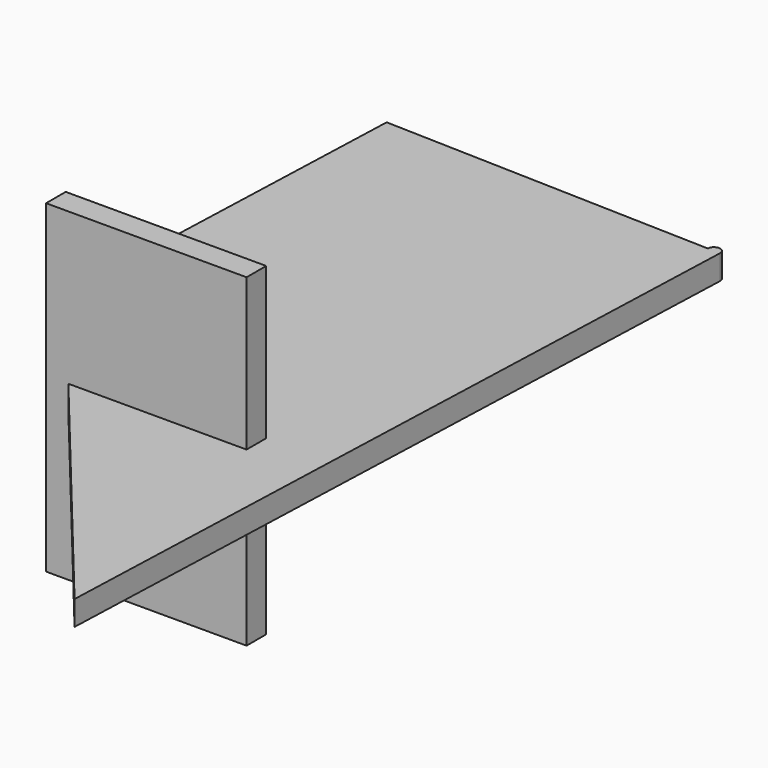
from build123d import *

# Parameters (mm, degrees)
F2_DEPTH = 25
F3_W     = 204.2875885963
F3_H     = 330.4814696312
F4_DEPTH = 25


with BuildPart() as f2:
    # F1 (on Top) → F2 (new body)
    with BuildSketch(Plane.XY):
        with BuildLine():
            Line((168.3422140292, 474.8379558081), (181.0361660289, 474.454610266))
            ThreePointArc((181.0361660289, 474.454610266), (174.8820955467, 481.0340797179), (168.3422140292, 474.8379558081))
        make_face()
        with BuildLine():
            Line((166.6445245232, 81.42426457), (181.0361660289, 474.454610266))
            Line((181.0361660289, 474.454610266), (168.3422140292, 474.8379558081))
            Line((168.3422140292, 474.8379558081), (-166.9943213011, 484.9648072356))
            Line((-166.9943213011, 484.9648072356), (-178.021518384, 183.8161801091))
            add(Edge.make_bspline(
                [(-178.021518384, 183.8161801091), (-126.121723234, 189.1373544028), (-5.2720297028, 157.9893070947), (124.2923755779, 80.293310388), (162.9702843725, 49.4019598786)],
                knots=[504.1665264406, 504.1665264406, 504.1665264406, 504.1665264406, 653.3978700476, 795.436226982, 795.436226982, 795.436226982, 795.436226982], degree=3))
            add(Edge.make_bspline(
                [(162.9702843725, 49.4019598786), (163.7914086642, 48.7461426667), (164.6014886785, 48.0934791624), (165.4002701181, 47.4441422338)],
                knots=[795.436226982, 795.436226982, 795.436226982, 795.436226982, 798.4516729787, 798.4516729787, 798.4516729787, 798.4516729787], degree=3))
            Line((165.4002701181, 47.4441422338), (166.6445245232, 81.42426457))
        make_face()
        with BuildLine():
            Line((163.474066231, -5.1597653413), (165.4002701181, 47.4441422338))
            add(Edge.make_bspline(
                [(162.9702843725, 49.4019598786), (163.7914086642, 48.7461426667), (164.6014886785, 48.0934791624), (165.4002701181, 47.4441422338)],
                knots=[795.436226982, 795.436226982, 795.436226982, 795.436226982, 798.4516729787, 798.4516729787, 798.4516729787, 798.4516729787], degree=3))
            Line((162.9702843725, 49.4019598786), (160.9759493271, -5.0625841432))
            add(Edge.make_bspline(
                [(163.474066231, -5.1597653413), (162.6521846932, -5.131062894), (161.8193790258, -5.0986033684), (160.9759493271, -5.0625841432)],
                knots=[958.9382746439, 958.9382746439, 958.9382746439, 958.9382746439, 961.7589781967, 961.7589781967, 961.7589781967, 961.7589781967], degree=3))
        make_face()
        with BuildLine():
            Line((160.9759493271, -5.0625841432), (162.9702843725, 49.4019598786))
            add(Edge.make_bspline(
                [(-178.021518384, 183.8161801091), (-126.121723234, 189.1373544028), (-5.2720297028, 157.9893070947), (124.2923755779, 80.293310388), (162.9702843725, 49.4019598786)],
                knots=[504.1665264406, 504.1665264406, 504.1665264406, 504.1665264406, 653.3978700476, 795.436226982, 795.436226982, 795.436226982, 795.436226982], degree=3))
            Line((-178.021518384, 183.8161801091), (-181.3042814193, 94.1651496755))
            Line((-181.3042814193, 94.1651496755), (-88.1747823589, -19.1265900522))
            add(Edge.make_bspline(
                [(160.9759493271, -5.0625841432), (121.4037743321, -3.3726281412), (19.2880670567, 12.0779258477), (-62.8138782039, -5.4855367148), (-88.1747823589, -19.1265900522)],
                knots=[961.7589781967, 961.7589781967, 961.7589781967, 961.7589781967, 1094.1012170077, 1176.4100957539, 1176.4100957539, 1176.4100957539, 1176.4100957539], degree=3))
        make_face()
        with BuildLine():
            Line((159.4487037703, -115.0909082779), (163.474066231, -5.1597653413))
            add(Edge.make_bspline(
                [(163.474066231, -5.1597653413), (162.6521846932, -5.131062894), (161.8193790258, -5.0986033684), (160.9759493271, -5.0625841432)],
                knots=[958.9382746439, 958.9382746439, 958.9382746439, 958.9382746439, 961.7589781967, 961.7589781967, 961.7589781967, 961.7589781967], degree=3))
            add(Edge.make_bspline(
                [(160.9759493271, -5.0625841432), (121.4037743321, -3.3726281412), (19.2880670567, 12.0779258477), (-62.8138782039, -5.4855367148), (-88.1747823589, -19.1265900522)],
                knots=[961.7589781967, 961.7589781967, 961.7589781967, 961.7589781967, 1094.1012170077, 1176.4100957539, 1176.4100957539, 1176.4100957539, 1176.4100957539], degree=3))
            Line((-88.1747823589, -19.1265900522), (152.2528830175, -311.6060811259))
            Line((152.2528830175, -311.6060811259), (155.8507933939, -213.3484947019))
            Line((155.8507933939, -213.3484947019), (159.4487037703, -115.0909082779))
        make_face()
    extrude(amount=F2_DEPTH)

    # F3 (on face) → F4 (join)
    with BuildSketch(Plane.XZ):
        with Locations((-3.8982927799, 14.3264830112)):
            Rectangle(F3_W, F3_H)
    extrude(amount=F4_DEPTH)


solid = f2.part
